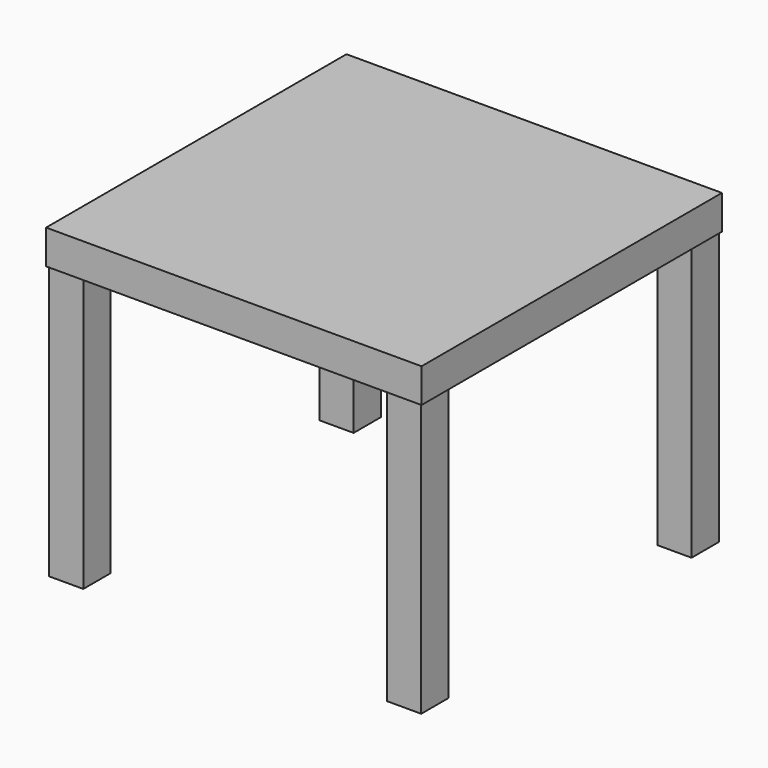
from build123d import *

# Parameters (mm, degrees)
F0_W          = 550
F0_H          = 550
F1_DEPTH      = 50
F0_W_2        = 50
F0_H_2        = 50
F2_DEPTH      = 50
F2_DEPTH_BACK = 400


with BuildPart() as f1:
    # F0 (on Top) → F1 (new body)
    with BuildSketch(Plane.XY):
        Rectangle(F0_W, F0_H)
        Polygon((222.5, 272.5), (272.5, 272.5), (272.5, 222.5), (272.5, -222.5), (272.5, -272.5), (222.5, -272.5), (-222.5, -272.5), (-272.5, -272.5), (-272.5, -222.5), (-272.5, 222.5), (-272.5, 272.5), (-222.5, 272.5), align=None, mode=Mode.SUBTRACT)
        Polygon((222.5, 222.5), (222.5, 272.5), (-222.5, 272.5), (-222.5, 222.5), (-272.5, 222.5), (-272.5, -222.5), (-222.5, -222.5), (-222.5, -272.5), (222.5, -272.5), (222.5, -222.5), (272.5, -222.5), (272.5, 222.5), align=None)
    extrude(amount=F1_DEPTH)

    # F0 (on Top) → F2 (join, two sides)
    with BuildSketch(Plane.XY) as f2_sk:
        with Locations((-247.5, -247.5)):
            Rectangle(F0_W_2, F0_H_2)
        with Locations((247.5, -247.5)):
            Rectangle(F0_W_2, F0_H_2)
        with Locations((247.5, 247.5)):
            Rectangle(F0_W_2, F0_H_2)
        with Locations((-247.5, 247.5)):
            Rectangle(F0_W_2, F0_H_2)
    extrude(amount=F2_DEPTH)
    extrude(f2_sk.sketch, amount=-F2_DEPTH_BACK)


solid = f1.part
